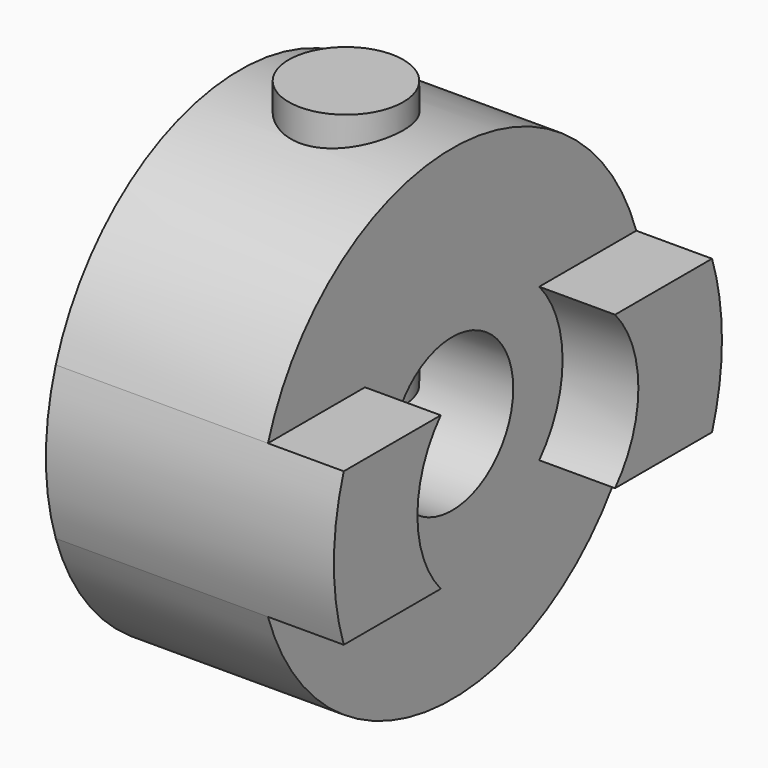
from build123d import *

# Parameters (mm, degrees)
F0_R     = 2
F1_DEPTH = 5.55625
F2_DEPTH = 1.984375
F3_R     = 1.5
F4_DEPTH = 7


# Not quite as in the source:
# - a length typed as a fraction of an inch, garbled in the dataset ("3 / 203.2 mm" for 3/8 in), is restored


with BuildPart() as f1:
    # F0 (on Right) → F1 (new body)
    with BuildSketch(Plane.YZ):
        with BuildLine():
            Line((2.851815, 2), (6.026815, 2))
            ThreePointArc((6.026815, 2), (0, 6.35), (-6.026815, 2))
            Line((-6.026815, 2), (-2.851815, 2))
            ThreePointArc((-2.851815, 2), (-3.615747, 0), (-2.851815, -2))
            Line((-2.851815, -2), (-6.026815, -2))
            ThreePointArc((-6.026815, -2), (0, -6.35), (6.026815, -2))
            Line((6.026815, -2), (2.851815, -2))
            ThreePointArc((2.851815, -2), (3.615747, 0), (2.851815, 2))
        make_face()
        Circle(F0_R, mode=Mode.SUBTRACT)
        with BuildLine():
            Line((-2.851815, 2), (-6.026815, 2))
            ThreePointArc((-6.026815, 2), (-6.35, 0), (-6.026815, -2))
            Line((-6.026815, -2), (-2.851815, -2))
            ThreePointArc((-2.851815, -2), (-3.615747, 0), (-2.851815, 2))
        make_face()
        with BuildLine():
            ThreePointArc((6.026815, -2), (6.268683, -1.012972), (6.35, 0))
            ThreePointArc((6.35, 0), (6.268683, 1.012972), (6.026815, 2))
            Line((6.026815, 2), (2.851815, 2))
            ThreePointArc((2.851815, 2), (3.615747, 0), (2.851815, -2))
            Line((2.851815, -2), (6.026815, -2))
        make_face()
    extrude(amount=-F1_DEPTH)

    # F0 (on Right) → F2 (join)
    with BuildSketch(Plane.YZ):
        with BuildLine():
            Line((-2.851815, 2), (-6.026815, 2))
            ThreePointArc((-6.026815, 2), (-6.35, 0), (-6.026815, -2))
            Line((-6.026815, -2), (-2.851815, -2))
            ThreePointArc((-2.851815, -2), (-3.615747, 0), (-2.851815, 2))
        make_face()
        with BuildLine():
            ThreePointArc((6.026815, -2), (6.268683, -1.012972), (6.35, 0))
            ThreePointArc((6.35, 0), (6.268683, 1.012972), (6.026815, 2))
            Line((6.026815, 2), (2.851815, 2))
            ThreePointArc((2.851815, 2), (3.615747, 0), (2.851815, -2))
            Line((2.851815, -2), (6.026815, -2))
        make_face()
    extrude(amount=F2_DEPTH)

    # F3 (on Top) → F4 (join)
    with BuildSketch(Plane.XY):
        with Locations((-2.778125, 0)):
            Circle(F3_R)
    extrude(amount=F4_DEPTH)


solid = f1.part
